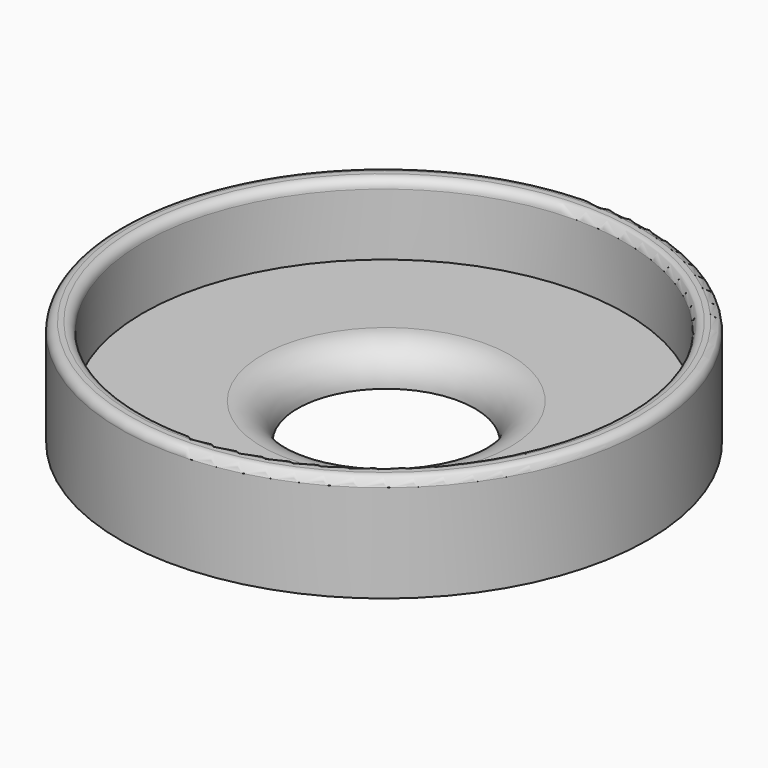
from build123d import *

# Parameters (mm, degrees)
F0_R     = 34
F0_R_2   = 12.5
F1_DEPTH = 5
F0_R_3   = 37.2
F2_DEPTH = 15
F3_R     = 1.25
F4_R     = 4.99999


# Not quite as in the source:
# - a fillet or chamfer is up to 0.001 mm smaller than in the source, because OpenCascade refuses the exact size


with BuildPart() as f1:
    # F0 (on Top) → F1 (new body)
    with BuildSketch(Plane.XY):
        Circle(F0_R)
        with Locations((0, 0.3778987616)):
            Circle(F0_R_2, mode=Mode.SUBTRACT)
    extrude(amount=F1_DEPTH)

    # F0 (on Top) → F2 (join)
    with BuildSketch(Plane.XY):
        Circle(F0_R_3)
        Circle(F0_R, mode=Mode.SUBTRACT)
    extrude(amount=F2_DEPTH)

    # F3
    f3_edges = [f1.edges().sort_by_distance(p)[0] for p in [
        (-34, 0, 15),
        (-37.2, 0, 15),
    ]]
    fillet(f3_edges, radius=F3_R)

    # F4 (radius 5 in the source; OpenCascade refuses exactly that, so slightly less here)
    f4_edges = [f1.edges().sort_by_distance(p)[0] for p in [
        (-12.5, 0.377899, 5),
    ]]
    fillet(f4_edges, radius=F4_R)


solid = f1.part
